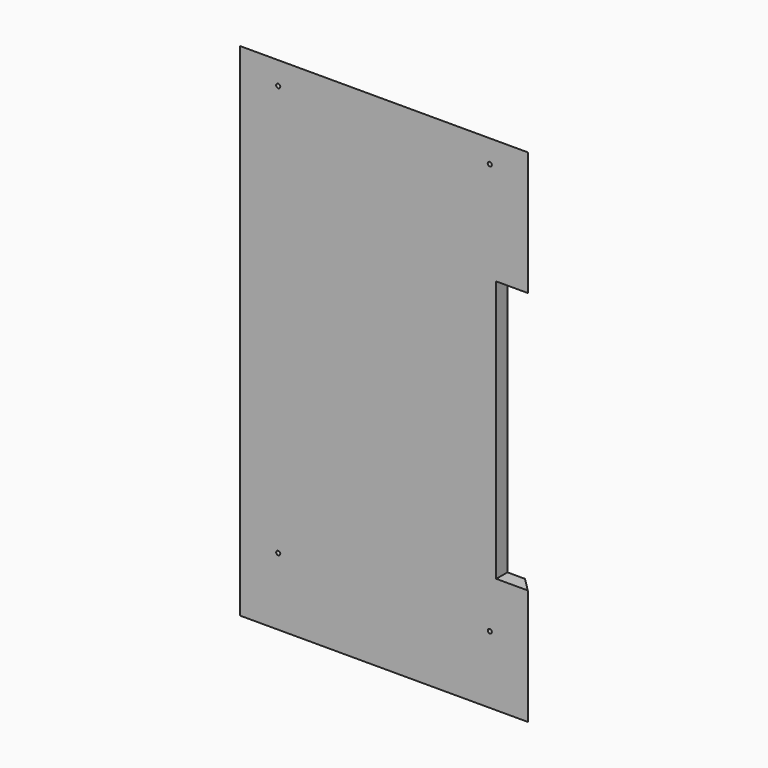
from build123d import *

# Parameters (mm, degrees)
F0_W     = 246
F0_H     = 429
F1_DEPTH = 12
F2_W     = 27
F2_H     = 224
F3_DEPTH = 25
F4_SIZE  = 11.99999
F6_D     = 3.5


# Not quite as in the source:
# - a fillet or chamfer is up to 0.001 mm smaller than in the source, because OpenCascade refuses the exact size


with BuildPart() as f1:
    # F0 (on Front) → F1 (new body)
    with BuildSketch(Plane.XZ):
        Rectangle(F0_W, F0_H)
    extrude(amount=F1_DEPTH)

    # F2 (on face) → F3 (cut)
    with BuildSketch(Plane(origin=(0, 0, 0), x_dir=(-1, 0, 0), z_dir=(0, 1, 0))):
        with Locations((-109.5, -3.5)):
            Rectangle(F2_W, F2_H)
    extrude(amount=-F3_DEPTH, mode=Mode.SUBTRACT)

    # F4 (size 12 in the source; OpenCascade refuses exactly that, so slightly less here)
    f4_edges = [f1.edges().sort_by_distance(p)[0] for p in [
        (0, 0, 214.5),
        (-123, 0, 0),
        (123, 0, 161.5),
        (123, 0, -165),
    ]]
    chamfer(f4_edges, length=F4_SIZE)

    # F6 (through all)
    with Locations(Plane.XZ.offset(12)):
        with Locations((-90.5, 195), (90.5, 195), (90.5, -156.8), (-90.5, -156.8)):
            Hole(F6_D / 2)


solid = f1.part
